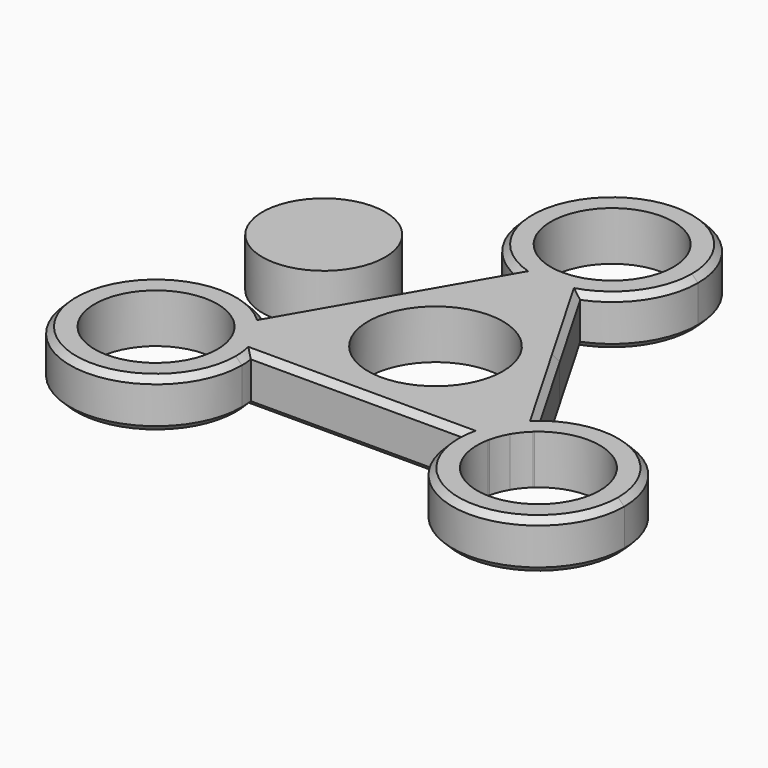
from build123d import *

# Parameters (mm, degrees)
F0_R     = 16
F0_R_2   = 11
F3_DEPTH = 8
F1_R     = 10
F4_DEPTH = 8
F5_DEPTH = 8
F6_SIZE  = 1


# Not quite as in the source:
# - a feature names something its author has since deleted; it is built from what else it names


with BuildPart() as f3:
    # F0 (on Top) → F3 (new body)
    with BuildSketch(Plane.XY):
        Circle(F0_R)
        Circle(F0_R_2, mode=Mode.SUBTRACT)
    extrude(amount=F3_DEPTH)

    # F2 (on Top) → F5 (join)
    with BuildSketch(Plane.XY):
        with BuildLine():
            Line((-21.3789555651, -16), (-17.3205080757, -16))
            ThreePointArc((-17.3205080757, -16), (-17.3669363919, -15.7011951683), (-17.4198074798, -15.4034627985))
            add(Edge.make_bspline(
                [(-21.4234698184, -15.7931207247), (-20.0285376046, -15.6036170386), (-18.6973308898, -15.4789767493), (-17.4198074798, -15.4034627985)],
                knots=[0.1245766513, 0.1245766513, 0.1245766513, 0.1245766513, 0.1837378076, 0.1837378076, 0.1837378076, 0.1837378076], degree=3))
            ThreePointArc((-21.4234698184, -15.7931207247), (-21.4006654441, -15.896442611), (-21.3789555651, -16))
        make_face()
        with BuildLine():
            ThreePointArc((-17.4198074798, -15.4034627985), (-18.0502184878, -13.1327779123), (-19.0525588833, -11))
            Line((-19.0525588833, -11), (-22.5166604984, -13))
            ThreePointArc((-22.5166604984, -13), (-21.8647474248, -14.3553403879), (-21.4234698184, -15.7931207247))
            add(Edge.make_bspline(
                [(-21.4234698184, -15.7931207247), (-20.0285376046, -15.6036170386), (-18.6973308898, -15.4789767493), (-17.4198074798, -15.4034627985)],
                knots=[0.1245766513, 0.1245766513, 0.1245766513, 0.1245766513, 0.1837378076, 0.1837378076, 0.1837378076, 0.1837378076], degree=3))
        make_face()
        with BuildLine():
            ThreePointArc((-19.0525588833, -11), (-20.3984285382, -9.0655587981), (-22.0496938297, -7.3842644073))
            add(Edge.make_bspline(
                [(-24.3889786618, -10.6567087376), (-23.5273975486, -9.5434138469), (-22.7538525344, -8.4528751589), (-22.0496938297, -7.3842644073)],
                knots=[0.1245766513, 0.1245766513, 0.1245766513, 0.1245766513, 0.1837378076, 0.1837378076, 0.1837378076, 0.1837378076], degree=3))
            ThreePointArc((-24.3889786618, -10.6567087376), (-23.3644631683, -11.7577565232), (-22.5166604984, -13))
            Line((-22.5166604984, -13), (-19.0525588833, -11))
        make_face()
        with BuildLine():
            ThreePointArc((-22.0496938297, -7.3842644073), (-22.2811020815, -7.1896105172), (-22.5166604984, -7))
            Line((-22.5166604984, -7), (-24.5458842431, -10.5147186258))
            ThreePointArc((-24.5458842431, -10.5147186258), (-24.467055853, -10.585298627), (-24.3889786618, -10.6567087376))
            add(Edge.make_bspline(
                [(-24.3889786618, -10.6567087376), (-23.5273975486, -9.5434138469), (-22.7538525344, -8.4528751589), (-22.0496938297, -7.3842644073)],
                knots=[0.1245766513, 0.1245766513, 0.1245766513, 0.1245766513, 0.1837378076, 0.1837378076, 0.1837378076, 0.1837378076], degree=3))
        make_face()
        with BuildLine():
            Line((-24.5458842431, -10.5147186258), (-22.5166604984, -7))
            ThreePointArc((-22.5166604984, -7), (-43.7714283524, -24.1137731177), (-17.1769145362, -18))
            ThreePointArc((-17.1769145362, -18), (-17.2128590643, -16.9974259249), (-17.3205080757, -16))
            Line((-17.3205080757, -16), (-21.3789555651, -16))
            ThreePointArc((-21.3789555651, -16), (-21.2275530062, -16.9949103799), (-21.1769145362, -18))
            ThreePointArc((-21.1769145362, -18), (-40.2958591827, -22.104247621), (-24.5458842431, -10.5147186258))
        make_face()
        with BuildLine():
            ThreePointArc((-2.9655088434, 26.4498294623), (-3.0663904088, 26.481741238), (-3.166928678, 26.5147186258))
            Line((-3.166928678, 26.5147186258), (-5.1961524227, 23))
            ThreePointArc((-5.1961524227, 23), (-4.9141656896, 22.8908056855), (-4.6298863498, 22.7877272058))
            add(Edge.make_bspline(
                [(-4.6298863498, 22.7877272058), (-4.0565216445, 23.9318519082), (-3.498859944, 25.1470308855), (-2.9655088434, 26.4498294623)],
                knots=[0.8162621924, 0.8162621924, 0.8162621924, 0.8162621924, 0.8754233487, 0.8754233487, 0.8754233487, 0.8754233487], degree=3))
        make_face()
        with BuildLine():
            Line((0, 22), (0, 26))
            ThreePointArc((0, 26), (-1.4997157435, 26.1130969111), (-2.9655088434, 26.4498294623))
            add(Edge.make_bspline(
                [(-4.6298863498, 22.7877272058), (-4.0565216445, 23.9318519082), (-3.498859944, 25.1470308855), (-2.9655088434, 26.4498294623)],
                knots=[0.8162621924, 0.8162621924, 0.8162621924, 0.8162621924, 0.8754233487, 0.8754233487, 0.8754233487, 0.8754233487], degree=3))
            ThreePointArc((-4.6298863498, 22.7877272058), (-2.3482100504, 22.1983367104), (0, 22))
        make_face()
        with BuildLine():
            ThreePointArc((2.9655088434, 26.4498294623), (1.4997157435, 26.1130969111), (0, 26))
            Line((0, 26), (0, 22))
            ThreePointArc((0, 22), (2.3482100504, 22.1983367104), (4.6298863498, 22.7877272058))
            add(Edge.make_bspline(
                [(2.9655088434, 26.4498294623), (3.498859944, 25.1470308855), (4.0565216445, 23.9318519082), (4.6298863498, 22.7877272058)],
                knots=[0.1245766513, 0.1245766513, 0.1245766513, 0.1245766513, 0.1837378076, 0.1837378076, 0.1837378076, 0.1837378076], degree=3))
        make_face()
        with BuildLine():
            Line((5.1961524227, 23), (3.166928678, 26.5147186258))
            ThreePointArc((3.166928678, 26.5147186258), (3.0663904088, 26.481741238), (2.9655088434, 26.4498294623))
            add(Edge.make_bspline(
                [(2.9655088434, 26.4498294623), (3.498859944, 25.1470308855), (4.0565216445, 23.9318519082), (4.6298863498, 22.7877272058)],
                knots=[0.1245766513, 0.1245766513, 0.1245766513, 0.1245766513, 0.1837378076, 0.1837378076, 0.1837378076, 0.1837378076], degree=3))
            ThreePointArc((4.6298863498, 22.7877272058), (4.9141656896, 22.8908056855), (5.1961524227, 23))
        make_face()
        with BuildLine():
            ThreePointArc((10, 36), (8.1138550264, 30.1548860909), (3.166928678, 26.5147186258))
            Line((3.166928678, 26.5147186258), (5.1961524227, 23))
            ThreePointArc((5.1961524227, 23), (11.591939741, 28.1497176458), (14, 36))
            ThreePointArc((14, 36), (-7.8502823542, 47.591939741), (-5.1961524227, 23))
            Line((-5.1961524227, 23), (-3.166928678, 26.5147186258))
            ThreePointArc((-3.166928678, 26.5147186258), (-5.8451139091, 44.1138550264), (10, 36))
        make_face()
        with BuildLine():
            Line((24.5458842431, -10.5147186258), (22.5166604984, -7))
            ThreePointArc((22.5166604984, -7), (22.2811020815, -7.1896105172), (22.0496938297, -7.3842644073))
            add(Edge.make_bspline(
                [(22.0496938297, -7.3842644073), (22.7538525344, -8.4528751589), (23.5273975486, -9.5434138469), (24.3889786618, -10.6567087376)],
                knots=[0.8162621924, 0.8162621924, 0.8162621924, 0.8162621924, 0.8754233487, 0.8754233487, 0.8754233487, 0.8754233487], degree=3))
            ThreePointArc((24.3889786618, -10.6567087376), (24.467055853, -10.585298627), (24.5458842431, -10.5147186258))
        make_face()
        with BuildLine():
            add(Edge.make_bspline(
                [(22.0496938297, -7.3842644073), (22.7538525344, -8.4528751589), (23.5273975486, -9.5434138469), (24.3889786618, -10.6567087376)],
                knots=[0.8162621924, 0.8162621924, 0.8162621924, 0.8162621924, 0.8754233487, 0.8754233487, 0.8754233487, 0.8754233487], degree=3))
            ThreePointArc((22.0496938297, -7.3842644073), (20.3984285382, -9.0655587981), (19.0525588833, -11))
            Line((19.0525588833, -11), (22.5166604984, -13))
            ThreePointArc((22.5166604984, -13), (23.3644631683, -11.7577565232), (24.3889786618, -10.6567087376))
        make_face()
        with BuildLine():
            Line((22.5166604984, -13), (19.0525588833, -11))
            ThreePointArc((19.0525588833, -11), (18.0502184878, -13.1327779123), (17.4198074798, -15.4034627985))
            add(Edge.make_bspline(
                [(17.4198074798, -15.4034627985), (18.6973308898, -15.4789767493), (20.0285376046, -15.6036170386), (21.4234698184, -15.7931207247)],
                knots=[0.8162621924, 0.8162621924, 0.8162621924, 0.8162621924, 0.8754233487, 0.8754233487, 0.8754233487, 0.8754233487], degree=3))
            ThreePointArc((21.4234698184, -15.7931207247), (21.8647474248, -14.3553403879), (22.5166604984, -13))
        make_face()
        with BuildLine():
            ThreePointArc((17.4198074798, -15.4034627985), (17.3669363919, -15.7011951683), (17.3205080757, -16))
            Line((17.3205080757, -16), (21.3789555651, -16))
            ThreePointArc((21.3789555651, -16), (21.4006654441, -15.896442611), (21.4234698184, -15.7931207247))
            add(Edge.make_bspline(
                [(17.4198074798, -15.4034627985), (18.6973308898, -15.4789767493), (20.0285376046, -15.6036170386), (21.4234698184, -15.7931207247)],
                knots=[0.8162621924, 0.8162621924, 0.8162621924, 0.8162621924, 0.8754233487, 0.8754233487, 0.8754233487, 0.8754233487], degree=3))
        make_face()
        with BuildLine():
            ThreePointArc((45.1769145362, -18), (37.290687654, -5.4054861839), (22.5166604984, -7))
            Line((22.5166604984, -7), (24.5458842431, -10.5147186258))
            ThreePointArc((24.5458842431, -10.5147186258), (35.2811621572, -8.8810553535), (41.1769145362, -18))
            ThreePointArc((41.1769145362, -18), (30.1718249162, -27.9493615301), (21.3789555651, -16))
            Line((21.3789555651, -16), (17.3205080757, -16))
            ThreePointArc((17.3205080757, -16), (30.1743404611, -31.964055472), (45.1769145362, -18))
        make_face()
        with BuildLine():
            ThreePointArc((-4.6298863498, 22.7877272058), (-4.9141656896, 22.8908056855), (-5.1961524227, 23))
            Line((-5.1961524227, 23), (-13.8564064606, 8))
            add(Edge.make_bspline(
                [(-13.8564064606, 8), (-11.2087925627, 12.5858017899), (-7.6949646898, 16.671494708), (-4.6298863498, 22.7877272058)],
                knots=[0.5, 0.5, 0.5, 0.5, 0.8162621924, 0.8162621924, 0.8162621924, 0.8162621924], degree=3))
        make_face()
        with BuildLine():
            Line((13.8564064606, 8), (5.1961524227, 23))
            ThreePointArc((5.1961524227, 23), (4.9141656896, 22.8908056855), (4.6298863498, 22.7877272058))
            add(Edge.make_bspline(
                [(4.6298863498, 22.7877272058), (7.6949646898, 16.671494708), (11.2087925627, 12.5858017899), (13.8564064606, 8)],
                knots=[0.1837378076, 0.1837378076, 0.1837378076, 0.1837378076, 0.5, 0.5, 0.5, 0.5], degree=3))
        make_face()
        with BuildLine():
            add(Edge.make_bspline(
                [(-22.0496938297, -7.3842644073), (-18.2854202811, -1.6717124515), (-16.5040203584, 3.4141982101), (-13.8564064606, 8)],
                knots=[0.1837378076, 0.1837378076, 0.1837378076, 0.1837378076, 0.5, 0.5, 0.5, 0.5], degree=3))
            Line((-13.8564064606, 8), (-22.5166604984, -7))
            ThreePointArc((-22.5166604984, -7), (-22.2811020815, -7.1896105172), (-22.0496938297, -7.3842644073))
        make_face()
        with BuildLine():
            ThreePointArc((-13.8564064606, -8), (-16, 0), (-13.8564064606, 8))
            add(Edge.make_bspline(
                [(-22.0496938297, -7.3842644073), (-18.2854202811, -1.6717124515), (-16.5040203584, 3.4141982101), (-13.8564064606, 8)],
                knots=[0.1837378076, 0.1837378076, 0.1837378076, 0.1837378076, 0.5, 0.5, 0.5, 0.5], degree=3))
            ThreePointArc((-22.0496938297, -7.3842644073), (-20.3984285382, -9.0655587981), (-19.0525588833, -11))
            Line((-19.0525588833, -11), (-13.8564064606, -8))
        make_face()
        with BuildLine():
            ThreePointArc((0, -16), (-8, -13.8564064606), (-13.8564064606, -8))
            Line((-13.8564064606, -8), (-19.0525588833, -11))
            ThreePointArc((-19.0525588833, -11), (-18.0502184878, -13.1327779123), (-17.4198074798, -15.4034627985))
            add(Edge.make_bspline(
                [(-17.4198074798, -15.4034627985), (-10.5904555913, -14.9997822566), (-5.2952277957, -16), (0, -16)],
                knots=[0.1837378076, 0.1837378076, 0.1837378076, 0.1837378076, 0.5, 0.5, 0.5, 0.5], degree=3))
        make_face()
        with BuildLine():
            Line((-17.3205080757, -16), (0, -16))
            add(Edge.make_bspline(
                [(-17.4198074798, -15.4034627985), (-10.5904555913, -14.9997822566), (-5.2952277957, -16), (0, -16)],
                knots=[0.1837378076, 0.1837378076, 0.1837378076, 0.1837378076, 0.5, 0.5, 0.5, 0.5], degree=3))
            ThreePointArc((-17.4198074798, -15.4034627985), (-17.3669363919, -15.7011951683), (-17.3205080757, -16))
        make_face()
        with BuildLine():
            Line((19.0525588833, -11), (13.8564064606, -8))
            ThreePointArc((13.8564064606, -8), (8, -13.8564064606), (0, -16))
            add(Edge.make_bspline(
                [(0, -16), (5.2952277957, -16), (10.5904555913, -14.9997822566), (17.4198074798, -15.4034627985)],
                knots=[0.5, 0.5, 0.5, 0.5, 0.8162621924, 0.8162621924, 0.8162621924, 0.8162621924], degree=3))
            ThreePointArc((17.4198074798, -15.4034627985), (18.0502184878, -13.1327779123), (19.0525588833, -11))
        make_face()
        with BuildLine():
            add(Edge.make_bspline(
                [(0, -16), (5.2952277957, -16), (10.5904555913, -14.9997822566), (17.4198074798, -15.4034627985)],
                knots=[0.5, 0.5, 0.5, 0.5, 0.8162621924, 0.8162621924, 0.8162621924, 0.8162621924], degree=3))
            Line((0, -16), (17.3205080757, -16))
            ThreePointArc((17.3205080757, -16), (17.3669363919, -15.7011951683), (17.4198074798, -15.4034627985))
        make_face()
        with BuildLine():
            add(Edge.make_bspline(
                [(13.8564064606, 8), (16.5040203584, 3.4141982101), (18.2854202811, -1.6717124515), (22.0496938297, -7.3842644073)],
                knots=[0.5, 0.5, 0.5, 0.5, 0.8162621924, 0.8162621924, 0.8162621924, 0.8162621924], degree=3))
            ThreePointArc((13.8564064606, 8), (15.4548132206, 4.1411047216), (16, 0))
            ThreePointArc((16, 0), (15.4548132206, -4.1411047216), (13.8564064606, -8))
            Line((13.8564064606, -8), (19.0525588833, -11))
            ThreePointArc((19.0525588833, -11), (20.3984285382, -9.0655587981), (22.0496938297, -7.3842644073))
        make_face()
        with BuildLine():
            Line((22.5166604984, -7), (13.8564064606, 8))
            add(Edge.make_bspline(
                [(13.8564064606, 8), (16.5040203584, 3.4141982101), (18.2854202811, -1.6717124515), (22.0496938297, -7.3842644073)],
                knots=[0.5, 0.5, 0.5, 0.5, 0.8162621924, 0.8162621924, 0.8162621924, 0.8162621924], degree=3))
            ThreePointArc((22.0496938297, -7.3842644073), (22.2811020815, -7.1896105172), (22.5166604984, -7))
        make_face()
        with BuildLine():
            Line((0, 16), (0, 22))
            ThreePointArc((0, 22), (-2.3482100504, 22.1983367104), (-4.6298863498, 22.7877272058))
            add(Edge.make_bspline(
                [(-13.8564064606, 8), (-11.2087925627, 12.5858017899), (-7.6949646898, 16.671494708), (-4.6298863498, 22.7877272058)],
                knots=[0.5, 0.5, 0.5, 0.5, 0.8162621924, 0.8162621924, 0.8162621924, 0.8162621924], degree=3))
            ThreePointArc((-13.8564064606, 8), (-8, 13.8564064606), (0, 16))
        make_face()
        with BuildLine():
            ThreePointArc((4.6298863498, 22.7877272058), (2.3482100504, 22.1983367104), (0, 22))
            Line((0, 22), (0, 16))
            ThreePointArc((0, 16), (8, 13.8564064606), (13.8564064606, 8))
            add(Edge.make_bspline(
                [(4.6298863498, 22.7877272058), (7.6949646898, 16.671494708), (11.2087925627, 12.5858017899), (13.8564064606, 8)],
                knots=[0.1837378076, 0.1837378076, 0.1837378076, 0.1837378076, 0.5, 0.5, 0.5, 0.5], degree=3))
        make_face()
    extrude(amount=F5_DEPTH)

    # F6
    f6_edges = [f3.edges().sort_by_distance(p)[0] for p in [
        (-43.30127, -25, 8),
        (-43.30127, -25, 0),
        (43.30127, -25, 8),
        (43.30127, -25, 0),
        (0, 50, 8),
        (0, 50, 0),
        (0, -16, 8),
        (-13.856406, 8, 8),
        (13.856406, 8, 8),
        (13.856406, 8, 0),
        (0, -16, 0),
        (-13.856406, 8, 0),
    ]]
    chamfer(f6_edges, length=F6_SIZE)


with BuildPart() as f4:
    # F1 (on Top) → F4 (new body)
    with BuildSketch(Plane.XY):
        with Locations((-60.5553910136, 57.5696118176)):
            Circle(F1_R)
    extrude(amount=F4_DEPTH)


with BuildPart() as f4_1:
    # F7: moved
    add(f4.part.moved(Location((30.2, -42.4, 0))))


solid = Compound([f3.part, f4_1.part])
